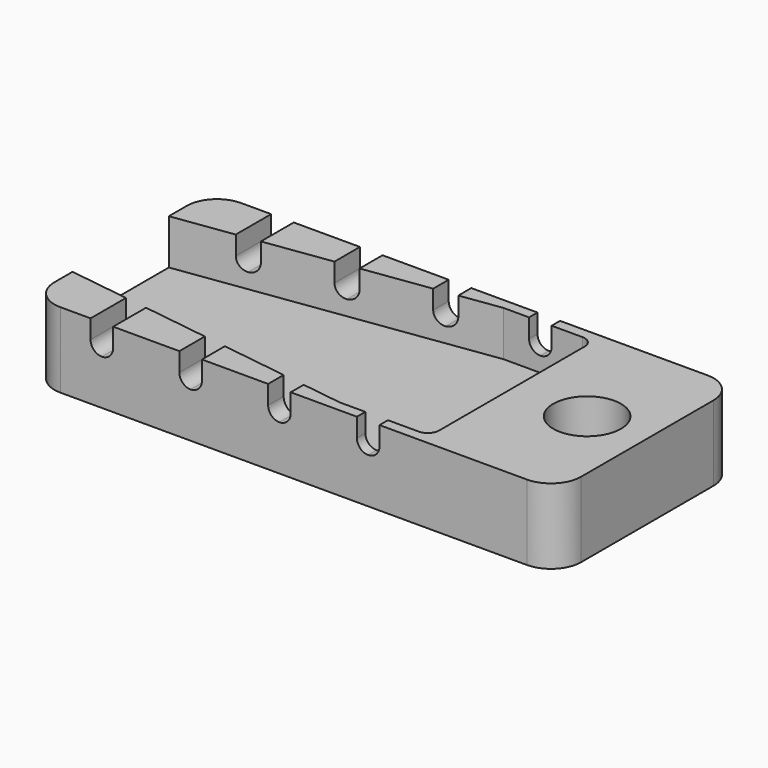
from build123d import *

# Parameters (mm, degrees)
F0_W     = 1.5
F0_H     = 0.7
F0_R     = 2.25
F0_H_2   = 13.6
F0_W_2   = 2.8
F1_DEPTH = 5
F2_DEPTH = 3
F3_DEPTH = 2
F4_R     = 0.74999
F5_R     = 2


# Not quite as in the source:
# - a fillet or chamfer is up to 0.001 mm smaller than in the source, because OpenCascade refuses the exact size


with BuildPart() as f1:
    # F0 (on Top) → F1 (new body)
    with BuildSketch(Plane.XY):
        Polygon((-18.8879279066, 7.5), (-22.8879279066, 7.5), (-22.8879279066, 4), (-18.8879279066, 4.56), align=None)
        Polygon((-17.3879279066, 7.5), (-18.8879279066, 7.5), (-18.8879279066, 4.56), (-17.3879279066, 4.77), align=None)
        Polygon((-18.8879279066, 4.56), (-22.8879279066, 4), (-22.8879279066, -4), (-18.8879279066, -4.56), align=None)
        Polygon((-12.9879279066, 7.5), (-17.3879279066, 7.5), (-17.3879279066, 4.77), (-12.9879279066, 5.386), align=None)
        Polygon((-18.8879279066, -4.56), (-22.8879279066, -4), (-22.8879279066, -7.5), (-18.8879279066, -7.5), align=None)
        Polygon((-11.4879279066, 7.5), (-12.9879279066, 7.5), (-12.9879279066, 5.386), (-11.4879279066, 5.596), align=None)
        Polygon((-17.3879279066, -4.77), (-18.8879279066, -4.56), (-18.8879279066, -7.5), (-17.3879279066, -7.5), align=None)
        Polygon((-7.0879279066, 7.5), (-11.4879279066, 7.5), (-11.4879279066, 5.596), (-7.0879279066, 6.212), align=None)
        Polygon((-12.9879279066, -5.386), (-17.3879279066, -4.77), (-17.3879279066, -7.5), (-12.9879279066, -7.5), align=None)
        Polygon((-5.5879279066, 7.5), (-7.0879279066, 7.5), (-7.0879279066, 6.212), (-5.5879279066, 6.422), align=None)
        Polygon((-11.4879279066, -5.596), (-12.9879279066, -5.386), (-12.9879279066, -7.5), (-11.4879279066, -7.5), align=None)
        Polygon((-1.1879279066, 7.5), (-5.5879279066, 7.5), (-5.5879279066, 6.422), (-2.8879279066, 6.8), (-1.1879279066, 6.8), align=None)
        Polygon((-7.0879279066, -6.212), (-11.4879279066, -5.596), (-11.4879279066, -7.5), (-7.0879279066, -7.5), align=None)
        with Locations((-0.4379279066, 7.15)):
            Rectangle(F0_W, F0_H)
        Polygon((-5.5879279066, -6.422), (-7.0879279066, -6.212), (-7.0879279066, -7.5), (-5.5879279066, -7.5), align=None)
        Polygon((12.1120720934, 7.5), (0.3120720934, 7.5), (0.3120720934, 6.8), (3.1120720934, 6.8), (3.1120720934, -6.8), (0.3120720934, -6.8), (0.3120720934, -7.5), (12.1120720934, -7.5), align=None)
        with Locations((8.1120720934, 0)):
            Circle(F0_R, mode=Mode.SUBTRACT)
        Polygon((-2.8879279066, -6.8), (-5.5879279066, -6.422), (-5.5879279066, -7.5), (-1.1879279066, -7.5), (-1.1879279066, -6.8), align=None)
        with Locations((-0.4379279066, -7.15)):
            Rectangle(F0_W, F0_H)
        with Locations((-0.4379279066, 0)):
            Rectangle(F0_W, F0_H_2)
        Polygon((-5.5879279066, 6.422), (-7.0879279066, 6.212), (-7.0879279066, -6.212), (-5.5879279066, -6.422), align=None)
        Polygon((-17.3879279066, 4.77), (-18.8879279066, 4.56), (-18.8879279066, -4.56), (-17.3879279066, -4.77), align=None)
        Polygon((-12.9879279066, 5.386), (-17.3879279066, 4.77), (-17.3879279066, -4.77), (-12.9879279066, -5.386), align=None)
        Polygon((-7.0879279066, 6.212), (-11.4879279066, 5.596), (-11.4879279066, -5.596), (-7.0879279066, -6.212), align=None)
        Polygon((-11.4879279066, 5.596), (-12.9879279066, 5.386), (-12.9879279066, -5.386), (-11.4879279066, -5.596), align=None)
        Polygon((-2.8879279066, 6.8), (-5.5879279066, 6.422), (-5.5879279066, -6.422), (-2.8879279066, -6.8), (-1.1879279066, -6.8), (-1.1879279066, 6.8), align=None)
        with Locations((1.7120720934, 0)):
            Rectangle(F0_W_2, F0_H_2)
    extrude(amount=-F1_DEPTH)

    # F0 (on Top) → F2 (cut)
    with BuildSketch(Plane.XY):
        Polygon((-18.8879279066, 4.56), (-22.8879279066, 4), (-22.8879279066, -4), (-18.8879279066, -4.56), align=None)
        Polygon((-17.3879279066, 4.77), (-18.8879279066, 4.56), (-18.8879279066, -4.56), (-17.3879279066, -4.77), align=None)
        Polygon((-12.9879279066, 5.386), (-17.3879279066, 4.77), (-17.3879279066, -4.77), (-12.9879279066, -5.386), align=None)
        Polygon((-11.4879279066, 5.596), (-12.9879279066, 5.386), (-12.9879279066, -5.386), (-11.4879279066, -5.596), align=None)
        Polygon((-7.0879279066, 6.212), (-11.4879279066, 5.596), (-11.4879279066, -5.596), (-7.0879279066, -6.212), align=None)
        Polygon((-5.5879279066, 6.422), (-7.0879279066, 6.212), (-7.0879279066, -6.212), (-5.5879279066, -6.422), align=None)
        Polygon((-2.8879279066, 6.8), (-5.5879279066, 6.422), (-5.5879279066, -6.422), (-2.8879279066, -6.8), (-1.1879279066, -6.8), (-1.1879279066, 6.8), align=None)
        with Locations((-0.4379279066, 0)):
            Rectangle(F0_W, F0_H_2)
        with Locations((1.7120720934, 0)):
            Rectangle(F0_W_2, F0_H_2)
    extrude(amount=-F2_DEPTH, mode=Mode.SUBTRACT)

    # F0 (on Top) → F3 (cut)
    with BuildSketch(Plane.XY):
        Polygon((-17.3879279066, 7.5), (-18.8879279066, 7.5), (-18.8879279066, 4.56), (-17.3879279066, 4.77), align=None)
        Polygon((-11.4879279066, 7.5), (-12.9879279066, 7.5), (-12.9879279066, 5.386), (-11.4879279066, 5.596), align=None)
        Polygon((-5.5879279066, 7.5), (-7.0879279066, 7.5), (-7.0879279066, 6.212), (-5.5879279066, 6.422), align=None)
        with Locations((-0.4379279066, -7.15)):
            Rectangle(F0_W, F0_H)
        Polygon((-17.3879279066, -4.77), (-18.8879279066, -4.56), (-18.8879279066, -7.5), (-17.3879279066, -7.5), align=None)
        Polygon((-11.4879279066, -5.596), (-12.9879279066, -5.386), (-12.9879279066, -7.5), (-11.4879279066, -7.5), align=None)
        Polygon((-5.5879279066, -6.422), (-7.0879279066, -6.212), (-7.0879279066, -7.5), (-5.5879279066, -7.5), align=None)
        with Locations((-0.4379279066, 7.15)):
            Rectangle(F0_W, F0_H)
    extrude(amount=-F3_DEPTH, mode=Mode.SUBTRACT)

    # F4 (radius 0.75 in the source; OpenCascade refuses exactly that, so slightly less here)
    f4_edges = [f1.edges().sort_by_distance(p)[0] for p in [
        (-17.387928, -6.135, -2),
        (-11.487928, -6.548, -2),
        (-5.587928, -6.961, -2),
        (0.312072, -7.15, -2),
        (-18.887928, -6.03, -2),
        (-12.987928, -6.443, -2),
        (-7.087928, -6.856, -2),
        (-1.187928, -7.15, -2),
        (-18.887928, 6.03, -2),
        (-12.987928, 6.443, -2),
        (-7.087928, 6.856, -2),
        (-1.187928, 7.15, -2),
        (-17.387928, 6.135, -2),
        (-11.487928, 6.548, -2),
        (-5.587928, 6.961, -2),
        (0.312072, 7.15, -2),
        (3.112072, 6.8, -1.5),
        (3.112072, -6.8, -1.5),
    ]]
    fillet(f4_edges, radius=F4_R)

    # F5
    f5_edges = [f1.edges().sort_by_distance(p)[0] for p in [
        (-22.887928, -7.5, -2.5),
        (-22.887928, 7.5, -2.5),
        (12.112072, -7.5, -2.5),
        (12.112072, 7.5, -2.5),
    ]]
    fillet(f5_edges, radius=F5_R)


solid = f1.part
